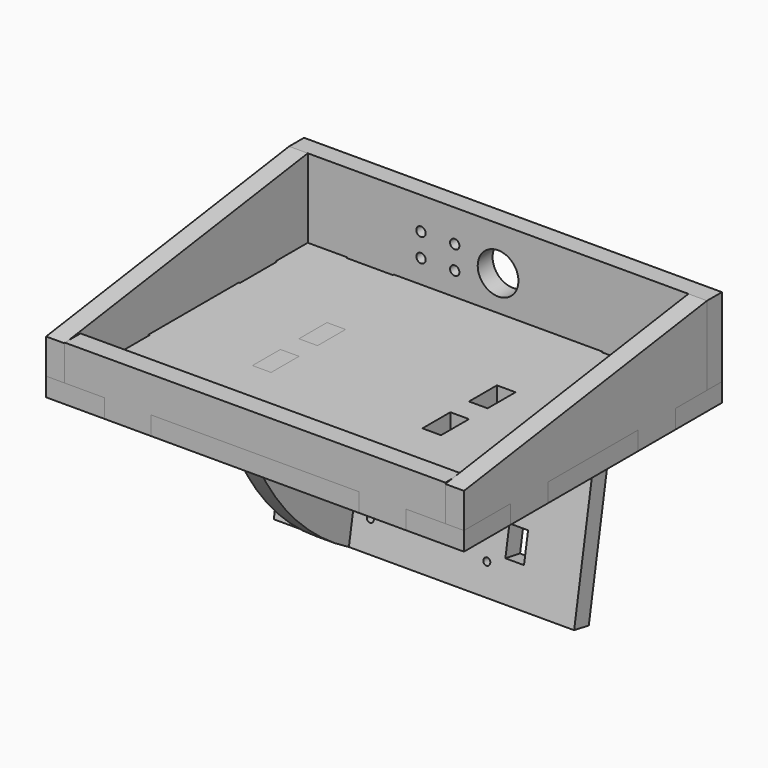
from build123d import *

# Parameters (mm, degrees)
F1_DEPTH  = 16
F2_W      = 40
F2_H      = 16
F3_DEPTH  = 16
F5_DEPTH  = 16
F7_DEPTH  = 16
F9_DEPTH  = 17
F10_R     = 17.5
F10_R_2   = 4
F11_DEPTH = 25
F12_W     = 16
F12_H     = 30
F13_DEPTH = 25
F14_W     = 30
F14_H     = 16
F15_DEPTH = 16
F16_W     = 258
F16_H     = 143.5460233889
F16_R     = 3
F16_W_2   = 16
F16_H_2   = 25
F17_DEPTH = 16


with BuildPart() as f1:
    # F0 (on Top) → F1 (new body)
    with BuildSketch(Plane.XY):
        Polygon((129.5, -138.5), (179.5, -138.5), (179.5, -88.5), (162.5, -88.5), (162.5, -48.5), (179.5, -48.5), (179.5, 48.5), (162.5, 48.5), (162.5, 88.5), (179.5, 88.5), (179.5, 138.5), (129.5, 138.5), (129.5, 121.5), (89.5, 121.5), (89.5, 138.5), (-89.5, 138.5), (-89.5, 121.5), (-129.5, 121.5), (-129.5, 138.5), (-179.5, 138.5), (-179.5, 88.5), (-162.5, 88.5), (-162.5, 48.5), (-179.5, 48.5), (-179.5, -48.5), (-162.5, -48.5), (-162.5, -88.5), (-179.5, -88.5), (-179.5, -138.5), (-129.5, -138.5), (-129.5, -121.5), (-89.5, -121.5), (-89.5, -138.5), (89.5, -138.5), (89.5, -121.5), (129.5, -121.5), align=None)
    extrude(amount=F1_DEPTH)

    # F12 (on face) → F13 (cut)
    with BuildSketch(Plane(origin=(0, 0, 0), x_dir=(1, 0, 0), z_dir=(0, 0, -1))):
        with Locations((73, -25)):
            Rectangle(F12_W, F12_H)
        with Locations((73, 25)):
            Rectangle(F12_W, F12_H)
        with Locations((-73, -25)):
            Rectangle(F12_W, F12_H)
        with Locations((-73, 25)):
            Rectangle(F12_W, F12_H)
    extrude(amount=-F13_DEPTH, mode=Mode.SUBTRACT)


with BuildPart() as f3:
    # F2 (on face) → F3 (new body)
    with BuildSketch(Plane(origin=(-179.5, 0, 0), x_dir=(0, -1, 0), z_dir=(-1, 0, 0))):
        with Locations((-68.5, 8)):
            Rectangle(F2_W, F2_H)
        with Locations((68.5, 8)):
            Rectangle(F2_W, F2_H)
        Polygon((-122.5, 16), (-88.5, 16), (-48.5, 16), (48.5, 16), (88.5, 16), (138.5, 16), (138.5, 46), (-122.5, 83.6895306859), align=None)
    extrude(amount=-F3_DEPTH)


with BuildPart() as f5:
    # F4 (on face) → F5 (new body)
    with BuildSketch(Plane(origin=(0, 138.5, 0), x_dir=(-1, 0, 0), z_dir=(0, 1, 0))):
        Polygon((129.5, 16), (179.5, 16), (179.5, 83.6895306859), (-179.5, 83.6895306859), (-179.5, 16), (-129.5, 16), (-129.5, 0), (-89.5, 0), (-89.5, 16), (89.3506407738, 16), (89.3506407738, 0), (129.5, 0), align=None)
    extrude(amount=-F5_DEPTH)

    # F10 (on face) → F11 (cut)
    with BuildSketch(Plane(origin=(0, 138.5, 0), x_dir=(-1, 0, 0), z_dir=(0, 1, 0))):
        with Locations((0, 46)):
            Circle(F10_R)
        with Locations((37.2249260545, 56)):
            Circle(F10_R_2)
        with Locations((66.2137439211, 56)):
            Circle(F10_R_2)
        with Locations((66.2137439211, 36)):
            Circle(F10_R_2)
        with Locations((37.2249260545, 36)):
            Circle(F10_R_2)
    extrude(amount=-F11_DEPTH, mode=Mode.SUBTRACT)


with BuildPart() as f7:
    # F6 (on face) → F7 (new body)
    with BuildSketch(Plane.YZ.offset(179.5)):
        Polygon((-138.5, 46), (-138.5, 16), (-88.5, 16), (-88.5, 0), (-48.5, 0), (-48.5, 16), (48.5, 16), (48.5, 0), (88.5, 0), (88.5, 16), (122.5, 16), (122.5, 83.6895306859), align=None)
    extrude(amount=-F7_DEPTH)


with BuildPart() as f9:
    # F8 (on face) → F9 (new body)
    with BuildSketch(Plane.XZ.offset(138.5)):
        Polygon((163.5, 47.0611862838), (-163.5, 46.5962067246), (-163.5, 16), (-129.5, 16), (-129.5, 0), (-89.5, 0), (-89.5, 16), (89.5, 16), (89.5, 0), (129.5, 0), (129.5, 16), (163.5, 16), align=None)
    extrude(amount=-F9_DEPTH)


with BuildPart() as f15:
    # F14 (on face) → F15 (new body)
    with BuildSketch(Plane.YZ.offset(-81)):
        with Locations((-25, 8)):
            Rectangle(F14_W, F14_H)
        Polygon((53.4488990207, -93.8659580783), (49.1076945791, -118.4861519036), (64.8646186273, -121.2645227463), (69.2058230689, -96.644328921), align=None)
        Polygon((62.9207125198, -40.1486343825), (58.5795080781, -64.7688282078), (74.3364321263, -67.5471990505), (78.677636568, -42.9270052252), align=None)
        with BuildLine():
            Line((-10, 0), (-40, 0))
            Line((-40, 0), (-73.0473920703, 0))
            ThreePointArc((-73.0473920703, 0), (-30.1908089692, -87.0038690918), (43.5509528937, -150))
            Line((43.5509528937, -150), (49.1076945791, -118.4861519036))
            Line((49.1076945791, -118.4861519036), (53.4488990207, -93.8659580783))
            Line((53.4488990207, -93.8659580783), (58.5795080781, -64.7688282078))
            Line((58.5795080781, -64.7688282078), (62.9207125198, -40.1486343825))
            Line((62.9207125198, -40.1486343825), (70, 0))
            Line((70, 0), (40, 0))
            Line((40, 0), (40, 16))
            Line((40, 16), (9.887823835, 16))
            Line((9.887823835, 16), (9.887823835, 0))
            Line((9.887823835, 0), (-10, 0))
        make_face()
    extrude(amount=F15_DEPTH)


with BuildPart() as f17:
    # F16 (on face) → F17 (new body)
    with BuildSketch(Plane(origin=(0, 67.8892417275, -11.9707050164), x_dir=(-1, 0, 0), z_dir=(0, 0.984807753, -0.1736481777))):
        with Locations((0.5, -68.3856076517)):
            Rectangle(F16_W, F16_H)
        with Locations((-50, -115.1586193462)):
            Circle(F16_R, mode=Mode.SUBTRACT)
        with Locations((-73, -95.6586193462)):
            Rectangle(F16_W_2, F16_H_2, mode=Mode.SUBTRACT)
        with Locations((50, -115.1586193462)):
            Circle(F16_R, mode=Mode.SUBTRACT)
        with Locations((73, -95.6586193462)):
            Rectangle(F16_W_2, F16_H_2, mode=Mode.SUBTRACT)
        with Locations((-73, -41.1125959573)):
            Rectangle(F16_W_2, F16_H_2, mode=Mode.SUBTRACT)
        with Locations((-50, -15.1586193462)):
            Circle(F16_R, mode=Mode.SUBTRACT)
        with Locations((73, -41.1125959573)):
            Rectangle(F16_W_2, F16_H_2, mode=Mode.SUBTRACT)
        with Locations((50, -15.1586193462)):
            Circle(F16_R, mode=Mode.SUBTRACT)
    extrude(amount=F17_DEPTH)


solid = Compound([f1.part, f3.part, f5.part, f7.part, f9.part, f15.part, f17.part])
